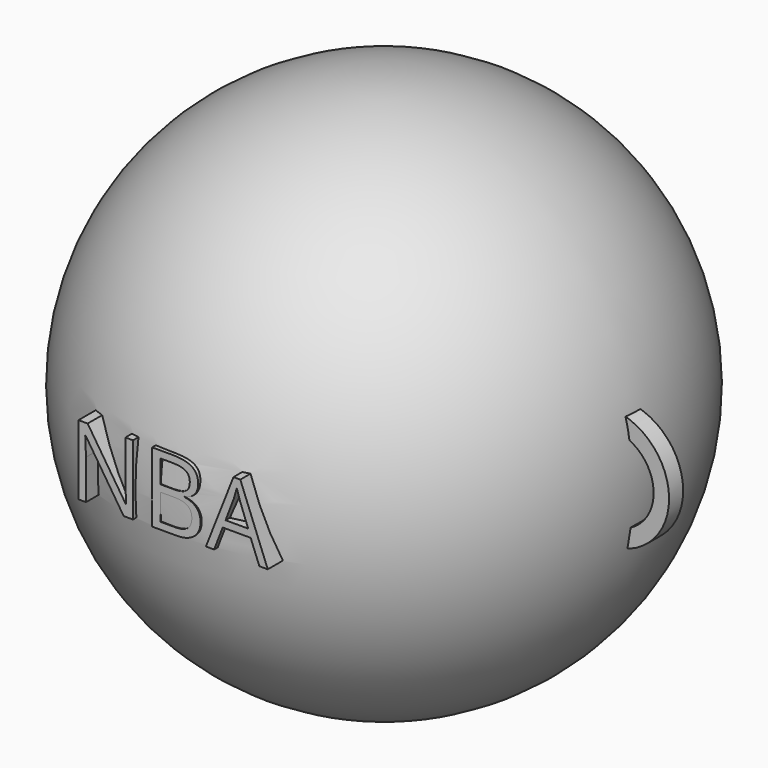
from build123d import *

# Parameters (mm, degrees)
F3_DEPTH     = 1.27
F4_TEXT_SIZE = 7.0555555556
F5_DEPTH     = 19.05


# Not quite as in the source:
# - Text() gives the source's letters only with a copy of the font that has no kerning and outlines rounded to 1/6400 em; it was checked with that copy


with BuildPart() as f1:
    # F0 (on Front) → F1 (revolve)
    with BuildSketch(Plane.XZ):
        with BuildLine():
            Line((0, 19.05), (0, -19.05))
            ThreePointArc((0, -19.05), (19.05, 0), (0, 19.05))
        make_face()
    revolve(axis=Axis((0, 0, 0), (0, 0, -1)))

    # F4 (on Front) → F5 (join)
    with BuildSketch(Plane.XZ):
        with Locations((-7.5076233862, -1.8064490085)):
            Text('NBA', F4_TEXT_SIZE, font='Open Sans', text_align=(TextAlign.LEFT, TextAlign.BOTTOM))
    extrude(amount=F5_DEPTH)


with BuildPart() as f3:
    # F2 (on Front) → F3 (new body)
    with BuildSketch(Plane.XZ):
        with BuildLine():
            Line((17.179331376, -2.832637867), (17.179331376, -4.1265841573))
            ThreePointArc((17.179331376, -4.1265841573), (21.5956483114, 0.2499984112), (17.179331376, 4.6265809797))
            Line((17.179331376, 4.6265809797), (17.179331376, 3.3326351549))
            ThreePointArc((17.179331376, 3.3326351549), (20.4828048478, 0.249998644), (17.179331376, -2.832637867))
        make_face()
    extrude(amount=F3_DEPTH)


solid = Compound([f1.part, f3.part])
